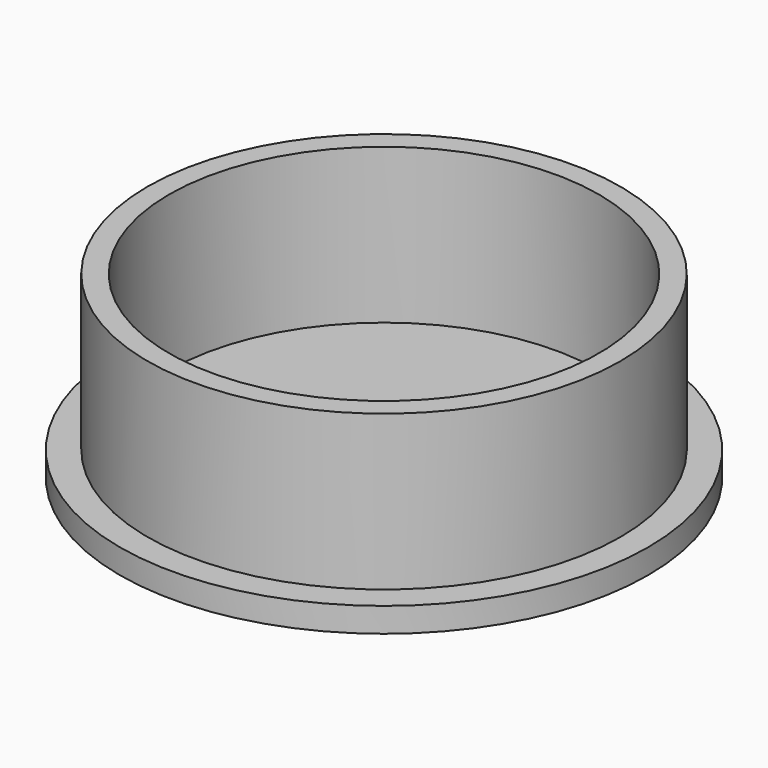
from build123d import *

# Parameters (mm, degrees)
F0_W   = 21.5
F0_H   = 4
F0_W_2 = 13.5
F0_W_3 = 3.492
F0_H_2 = 25.2048466533


# Not quite as in the source:
# - a feature names something its author has since deleted; it is built from what else it names


with BuildPart() as f1:
    # F0 (on Front) → F1 (revolve)
    with BuildSketch(Plane.XZ):
        with Locations((-59.25, -12.4232914925)):
            Rectangle(F0_W, F0_H)
        with Locations((-41.75, -12.4232914925)):
            Rectangle(F0_W_2, F0_H)
        with Locations((-71.746, 2.1791318342)):
            Rectangle(F0_W_3, F0_H_2)
        Polygon((-78, -14.4232914925), (-70, -14.4232914925), (-70, -10.4232914925), (-73.492, -10.4232914925), (-74, -10.4232914925), (-78, -10.4232914925), align=None)
    revolve(axis=Axis((-35, 0, -12.4232914925), (0, 0, 1)))


solid = f1.part
